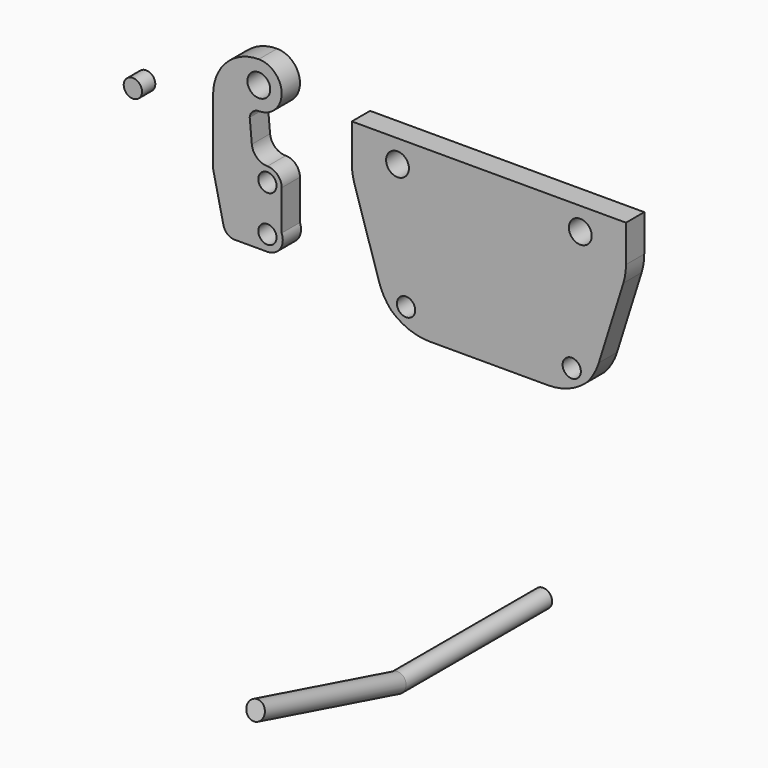
from build123d import *

# Parameters (mm, degrees)
F1_DEPTH    = 3.175
F2_D        = 3.175
F2_DEPTH    = 25.4
F2_TIP      = 0.9538662327
F3_D        = 2.54
F3_DEPTH    = 25.4
F3_TIP      = 0.7630929862
F5_DEPTH    = 3.175
F6_D        = 3.175
F6_DEPTH    = 25.4
F6_TIP      = 0.9538662327
F7_D        = 2.54
F7_DEPTH    = 25.4
F7_TIP      = 0.7630929862
F8_T1_DEPTH = 19.6141007567
F8_T3_DEPTH = 12.9058575482
F8_T5_DEPTH = 9.2647678202
F9_R        = 1.27
F10_DEPTH   = 2.3090909091
F11_R       = 1.27


# Not quite as in the source:
# - a fillet or chamfer that OpenCascade refuses, or shapes differently, is made with other operations: its cross-section is extruded or revolved along the edge and cut away or added


with BuildPart() as f1:
    # F0 (on Front) → F1 (new body)
    with BuildSketch(Plane.XZ):
        with BuildLine():
            ThreePointArc((-40.7624131311, 45.5551980838), (-40.3604208215, 46.3926978741), (-39.4958033942, 46.7324631164))
            ThreePointArc((-39.4958033942, 46.7324631164), (-36.3208033942, 49.9074631164), (-39.4958033942, 53.0824631164))
            ThreePointArc((-39.4958033942, 53.0824631164), (-43.9859314547, 51.222591177), (-45.8458033942, 46.7324631164))
            Line((-45.8458033942, 46.7324631164), (-45.8458033942, 37.5822147164))
            Line((-45.8458033942, 37.5822147164), (-44.4046161923, 31.1511978093))
            ThreePointArc((-44.4046161923, 31.1511978093), (-43.8477734395, 30.2591434316), (-42.8555409547, 29.9108482117))
            Line((-42.8555409547, 29.9108482117), (-38.3051783942, 29.9108482117))
            ThreePointArc((-38.3051783942, 29.9108482117), (-36.5353982281, 30.8498925673), (-36.3208033942, 32.841845176))
            Line((-36.3208033942, 32.841845176), (-36.3208033942, 38.3980881164))
            ThreePointArc((-36.3208033942, 38.3980881164), (-36.9020133752, 39.8012531354), (-38.3051783942, 40.3824631164))
            ThreePointArc((-38.3051783942, 40.3824631164), (-39.7708205612, 40.950778212), (-40.4701995839, 42.3585985103))
            Line((-40.4701995839, 42.3585985103), (-40.7624131311, 45.5551980838))
        make_face()
    extrude(amount=-F1_DEPTH)

    # F2
    with Locations(Plane.XZ):
        with Locations((-39.4958033942, 49.9074631164)):
            Hole(F2_D / 2, depth=F2_DEPTH)
            with Locations((0, 0, -(F2_DEPTH + F2_TIP / 2))):  # 118° drill point
                Cone(0, F2_D / 2, F2_TIP, mode=Mode.SUBTRACT)

    # F3
    with Locations(Plane.XZ):
        with Locations((-38.3051783942, 38.3980881164), (-38.3051783942, 32.0480881164)):
            Hole(F3_D / 2, depth=F3_DEPTH)
            with Locations((0, 0, -(F3_DEPTH + F3_TIP / 2))):  # 118° drill point
                Cone(0, F3_D / 2, F3_TIP, mode=Mode.SUBTRACT)


with BuildPart() as f5:
    # F4 (on Front) → F5 (new body)
    with BuildSketch(Plane.XZ):
        Polygon((11.5262488782, 49.6812058449), (-26.5737511218, 49.6812058449), (-26.5737511218, 46.5062058449), (-26.5737511218, 43.3312058449), (-22.2081261218, 29.4405808449), (-19.0331261218, 26.2655808449), (3.9856238782, 26.2655808449), (7.1606238782, 29.4405808449), (11.5262488782, 43.3312058449), (11.5262488782, 46.5062058449), align=None)
    extrude(amount=-F5_DEPTH)

    # F6
    with Locations(Plane.XZ):
        with Locations((-20.2237511218, 46.5062058449), (5.1762488782, 46.5062058449)):
            Hole(F6_D / 2, depth=F6_DEPTH)
            with Locations((0, 0, -(F6_DEPTH + F6_TIP / 2))):  # 118° drill point
                Cone(0, F6_D / 2, F6_TIP, mode=Mode.SUBTRACT)

    # F7
    with Locations(Plane.XZ):
        with Locations((-19.0331261218, 29.4405808449), (3.9856238782, 29.4405808449)):
            Hole(F7_D / 2, depth=F7_DEPTH)
            with Locations((0, 0, -(F7_DEPTH + F7_TIP / 2))):  # 118° drill point
                Cone(0, F7_D / 2, F7_TIP, mode=Mode.SUBTRACT)

    # F8: fillet of radius 7.9375 on 6 edges, made by hand

    # F8_s2 → F8_t1 (cut)
    with BuildSketch(Plane.XZ.offset(-11.3945503783)):
        with BuildLine():
            ThreePointArc((6.3104638026, 28.5904207692), (3.7353534713, 26.8697870556), (0.6978037269, 26.2655808449))
            Line((0.6978037269, 26.2655808449), (3.9856238782, 26.2655808449))
            Line((3.9856238782, 26.2655808449), (6.3104638026, 28.5904207692))
        make_face()
        with BuildLine():
            ThreePointArc((-21.3579660461, 28.5904207692), (-18.7828557148, 26.8697870556), (-15.7453059704, 26.2655808449))
            Line((-15.7453059704, 26.2655808449), (-19.0331261218, 26.2655808449))
            Line((-19.0331261218, 26.2655808449), (-21.3579660461, 28.5904207692))
        make_face()
    extrude(amount=F8_T1_DEPTH, mode=Mode.SUBTRACT)

    # F8_s4 → F8_t3 (cut)
    with BuildSketch(Plane.XZ.offset(-8.0404287741)):
        with BuildLine():
            ThreePointArc((7.7441378587, 31.2972162371), (6.9595727284, 29.562454936), (5.7844728064, 28.0644297731))
            Line((5.7844728064, 28.0644297731), (7.1606238782, 29.4405808449))
            Line((7.1606238782, 29.4405808449), (7.7441378587, 31.2972162371))
        make_face()
        with BuildLine():
            ThreePointArc((-22.7916401022, 31.2972162371), (-22.0070749719, 29.562454936), (-20.8319750499, 28.0644297731))
            Line((-20.8319750499, 28.0644297731), (-22.2081261218, 29.4405808449))
            Line((-22.2081261218, 29.4405808449), (-22.7916401022, 31.2972162371))
        make_face()
    extrude(amount=F8_T3_DEPTH, mode=Mode.SUBTRACT)

    # F8_s6 → F8_t5 (cut)
    with BuildSketch(Plane.XZ.offset(-6.2198839101)):
        with BuildLine():
            ThreePointArc((11.5262488782, 44.5491594089), (11.434424023, 43.3452957233), (11.1610740061, 42.1692857973))
            Line((11.1610740061, 42.1692857973), (11.5262488782, 43.3312058449))
            Line((11.5262488782, 43.3312058449), (11.5262488782, 44.5491594089))
        make_face()
        with BuildLine():
            ThreePointArc((-26.5737511218, 44.5491594089), (-26.4819262665, 43.3452957233), (-26.2085762497, 42.1692857973))
            Line((-26.2085762497, 42.1692857973), (-26.5737511218, 43.3312058449))
            Line((-26.5737511218, 43.3312058449), (-26.5737511218, 44.5491594089))
        make_face()
    extrude(amount=F8_T5_DEPTH, mode=Mode.SUBTRACT)


with BuildPart() as f10:
    # F9 (on Front) → F10 (new body)
    with BuildSketch(Plane.XZ):
        with Locations((-55.1536940038, 45.372158289)):
            Circle(F9_R)
    extrude(amount=F10_DEPTH)


with BuildPart() as f13:
    # F13: sweep along a path in F12
    with BuildLine(Plane.YZ) as f13_path:
        Line((0, 0), (-25.4, 0))
        Line((-25.4, 0), (-49.9345159877, 6.5740037456))
    # F11 (on Front) → F13 (sweep)
    with BuildSketch(Plane.XZ):
        Circle(F11_R)
    sweep(path=f13_path.line, transition=Transition.RIGHT)


solid = Compound([f1.part, f5.part, f10.part, f13.part])
